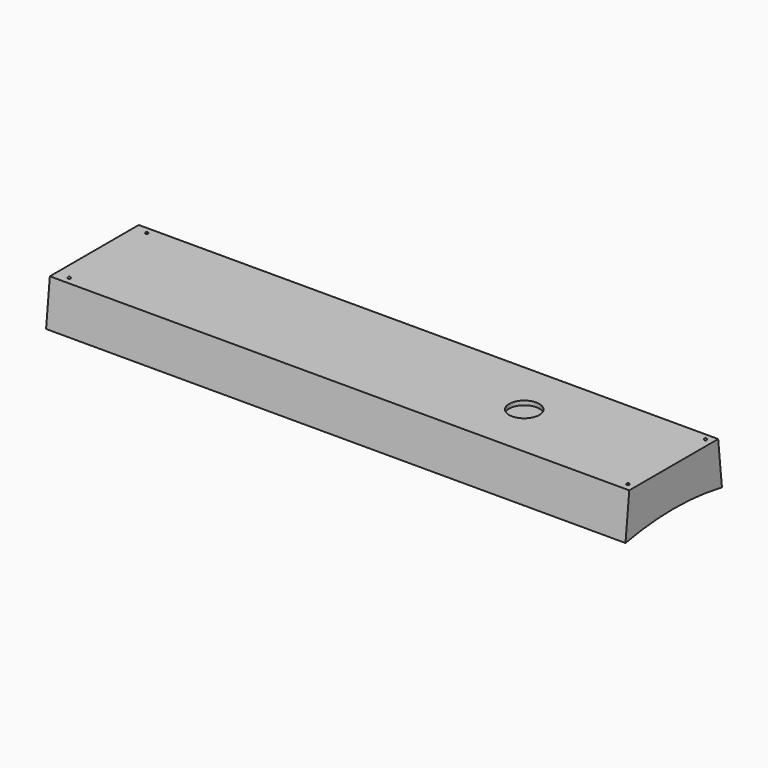
from build123d import *

# Parameters (mm, degrees)
F0_W          = 250
F0_H          = 52
F1_DEPTH      = 19.2
F2_SIZE2      = 2.017991
F2_SIZE       = 19.19999
F3_SIZE2      = 2.017991
F3_SIZE       = 19.19999
F4_R          = 6.5
F5_DEPTH      = 1.7951503396
F7_DEPTH      = 58.4841370583
F7_DEPTH_BACK = 301.5629071742
F8_R          = 0.55
F9_DEPTH      = 0.5
F10_R         = 0.49999
F11_R         = 0.49999
F12_R         = 13.25
F13_DEPTH     = 4
F14_W         = 21
F14_H         = 8
F14_H_2       = 8.9314985695
F15_DEPTH     = 4


# Not quite as in the source:
# - a fillet or chamfer is up to 0.001 mm smaller than in the source, because OpenCascade refuses the exact size


with BuildPart() as f1:
    # F0 (on Top) → F1 (new body)
    with BuildSketch(Plane.XY):
        with Locations((-1.4450065748, 26)):
            Rectangle(F0_W, F0_H)
    extrude(amount=F1_DEPTH)

    # F2 (size 19.2 and 2.0180013171 in the source; OpenCascade refuses exactly that, so slightly less here)
    f2_edges = [f1.edges().sort_by_distance(p)[0] for p in [
        (-1.445007, 52, 19.2),
    ]]
    f2_side = f1.faces().sort_by_distance((-1.445007, 52, 9.6))[0]
    chamfer(f2_edges, length=F2_SIZE, length2=F2_SIZE2, reference=f2_side)

    # F3 (size 19.2 and 2.0180013171 in the source; OpenCascade refuses exactly that, so slightly less here)
    f3_edges = [f1.edges().sort_by_distance(p)[0] for p in [
        (-1.445007, 0, 19.2),
    ]]
    f3_side = f1.faces().sort_by_distance((-1.445007, 0, 9.6))[0]
    chamfer(f3_edges, length=F3_SIZE, length2=F3_SIZE2, reference=f3_side)

    # F4 (on face) → F5 (cut)
    with BuildSketch(Plane.XY.offset(19.2)):
        with Locations((59.0549934252, 25.9999986829)):
            Circle(F4_R)
    extrude(amount=-F5_DEPTH, mode=Mode.SUBTRACT)

    # F6 (on face) → F7 (cut, two sides)
    with BuildSketch(Plane.YZ.offset(123.5549934252)) as f7_sk:
        Polygon((56.2664195895, -9.8316892982), (52, 0), (0, 0), (-4.1076340713, -9.8316892982), align=None)
        with BuildLine():
            Line((0, 0), (52, 0))
            ThreePointArc((52, 0), (26, 2.5), (0, 0))
        make_face()
    extrude(amount=F7_DEPTH, mode=Mode.SUBTRACT)
    extrude(f7_sk.sketch, amount=-F7_DEPTH_BACK, mode=Mode.SUBTRACT)

    # F8 (on face) → F9 (join)
    with BuildSketch(Plane.XY.offset(19.2)):
        with Locations((120.5049934252, 5.0680013171)):
            Circle(F8_R)
        with Locations((120.5049934252, 46.9319986829)):
            Circle(F8_R)
        with Locations((-120.5049934252, 5.0680013171)):
            Circle(F8_R)
        with Locations((-120.5049934252, 46.9319986829)):
            Circle(F8_R)
    extrude(amount=F9_DEPTH)

    # F10 (radius 0.5 in the source; OpenCascade refuses exactly that, so slightly less here)
    f10_edges = [f1.edges().sort_by_distance(p)[0] for p in [
        (119.954993, 5.068001, 19.7),
    ]]
    fillet(f10_edges, radius=F10_R)

    # F11 (radius 0.5 in the source; OpenCascade refuses exactly that, so slightly less here)
    f11_edges = [f1.edges().sort_by_distance(p)[0] for p in [
        (-121.054993, 5.068001, 19.7),
        (119.954993, 46.931999, 19.7),
        (-121.054993, 46.931999, 19.7),
    ]]
    fillet(f11_edges, radius=F11_R)

    # F12 (on Top) → F13 (cut)
    with BuildSketch(Plane.XY):
        with Locations((-35.1950065748, 26)):
            Circle(F12_R)
    extrude(amount=F13_DEPTH, mode=Mode.SUBTRACT)

    # F14 (on Top) → F15 (cut)
    with BuildSketch(Plane.XY):
        with Locations((48.0549934252, 34.5)):
            Rectangle(F14_W, F14_H)
        with Locations((48.0549934252, 17.9657492848)):
            Rectangle(F14_W, F14_H_2)
    extrude(amount=F15_DEPTH, mode=Mode.SUBTRACT)


solid = f1.part
